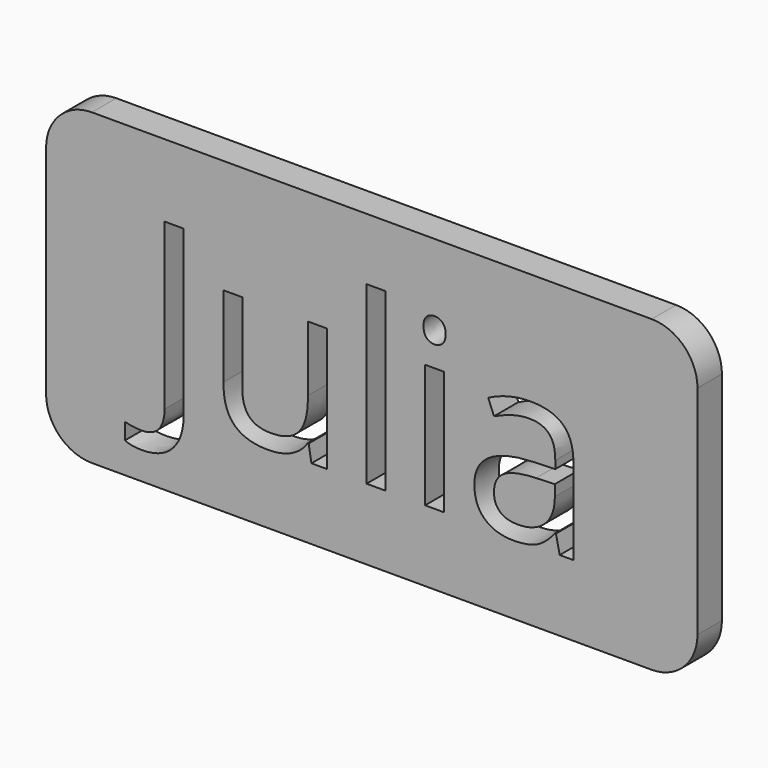
from build123d import *

# Parameters (mm, degrees)
F0_W         = 108.3454042673
F0_H         = 51.3498075306
F1_DEPTH     = 5.08
F2_R         = 7.62
F3_TEXT_SIZE = 38.4600794253
F4_DEPTH     = 5.081


# Not quite as in the source:
# - Text() gives the source's letters only with a copy of the font that has no kerning and outlines rounded to 1/6400 em; it was checked with that copy


with BuildPart() as f1:
    # F0 (on Front) → F1 (new body)
    with BuildSketch(Plane.XZ):
        with Locations((-4.4359788299, 1.7475094646)):
            Rectangle(F0_W, F0_H)
    extrude(amount=F1_DEPTH)

    # F2
    f2_edges = [f1.edges().sort_by_distance(p)[0] for p in [
        (-58.608681, -2.54, 27.422413),
        (-58.608681, -2.54, -23.927394),
        (49.736723, -2.54, 27.422413),
        (49.736723, -2.54, -23.927394),
    ]]
    fillet(f2_edges, radius=F2_R)

    # F3 (on face) → F4 (cut, through all)
    with BuildSketch(Plane.XZ.offset(5.08)):
        with Locations((-42.4778535962, -12.0981195942)):
            Text('Julia', F3_TEXT_SIZE, font='Open Sans', text_align=(TextAlign.LEFT, TextAlign.BOTTOM))
    extrude(amount=-F4_DEPTH, mode=Mode.SUBTRACT)


solid = f1.part
